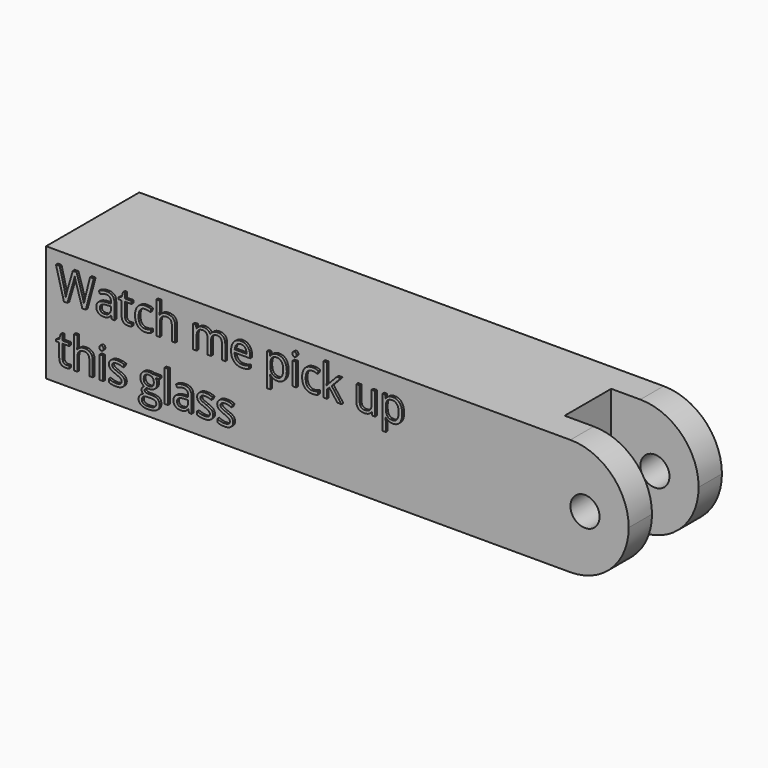
from build123d import *

# Parameters (mm, degrees)
F0_W         = 25.4
F0_H         = 25.4
F1_DEPTH     = 127
F2_W         = 19.05
F2_H         = 12.7
F3_DEPTH     = 25.4
F5_R         = 12.69999
F4_R         = 3.175
F6_DEPTH     = 29.3116
F7_W         = 12.7
F7_H         = 12.7
F8_DEPTH     = 76.2
F9_TEXT_SIZE = 9.1829702299
F10_DEPTH    = 0.508


# Not quite as in the source:
# - a fillet or chamfer is up to 0.001 mm smaller than in the source, because OpenCascade refuses the exact size
# - Text() gives the source's letters only with a copy of the font that has no kerning and outlines rounded to 1/6400 em; it was checked with that copy


with BuildPart() as f1:
    # F0 (on Right) → F1 (new body)
    with BuildSketch(Plane.YZ):
        Rectangle(F0_W, F0_H)
    extrude(amount=F1_DEPTH)

    # F2 (on face) → F3 (cut)
    with BuildSketch(Plane.XY.offset(12.7)):
        with Locations((117.475, 0)):
            Rectangle(F2_W, F2_H)
    extrude(amount=-F3_DEPTH, mode=Mode.SUBTRACT)

    # F5 (radius 12.7 in the source; OpenCascade refuses exactly that, so slightly less here)
    f5_edges = [f1.edges().sort_by_distance(p)[0] for p in [
        (127, -9.525, 12.7),
        (127, -9.525, -12.7),
        (127, 9.525, 12.7),
        (127, 9.525, -12.7),
    ]]
    fillet(f5_edges, radius=F5_R)

    # F4 (on face) → F6 (cut)
    with BuildSketch(Plane.XZ.offset(12.7)):
        with Locations((117.475, 0)):
            Circle(F4_R)
    extrude(amount=-F6_DEPTH, mode=Mode.SUBTRACT)

    # F7 (on face) → F8 (cut)
    with BuildSketch(Plane(origin=(0, 0, 0), x_dir=(0, -1, 0), z_dir=(-1, 0, 0))):
        Rectangle(F7_W, F7_H)
    extrude(amount=-F8_DEPTH, mode=Mode.SUBTRACT)

    # F9 (on face) → F10 (join)
    with BuildSketch(Plane.XZ.offset(12.7)):
        with Locations((2.4313907275, 3.6587857103)):
            Text('Watch me pick up', F9_TEXT_SIZE, font='Open Sans', text_align=(TextAlign.LEFT, TextAlign.BOTTOM))
        with Locations((2.4313907275, -8.8300538024)):
            Text('this glass', F9_TEXT_SIZE, font='Open Sans', text_align=(TextAlign.LEFT, TextAlign.BOTTOM))
    extrude(amount=F10_DEPTH)


solid = f1.part
